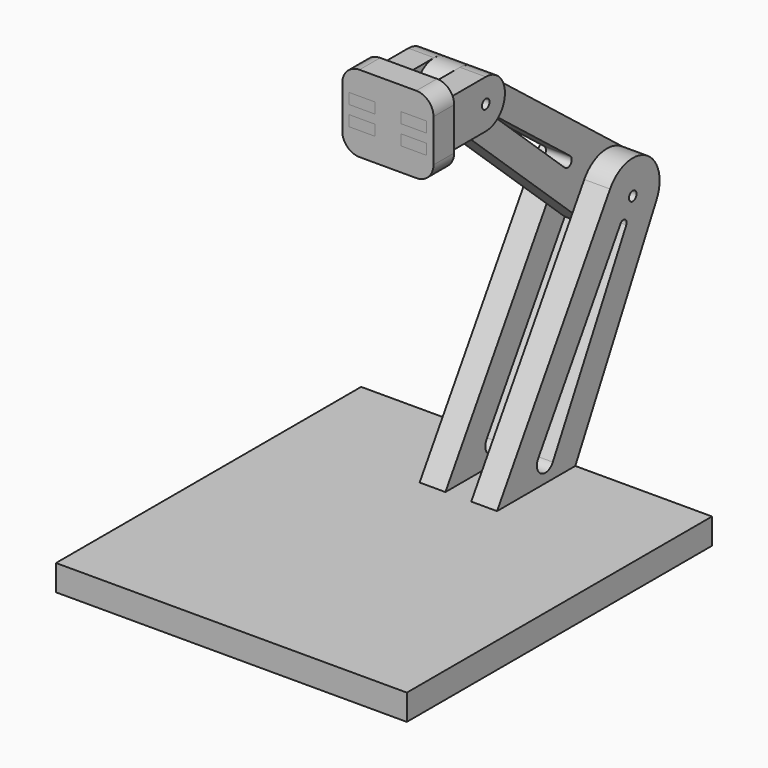
from build123d import *

# Parameters (mm, degrees)
F1_W      = 258.9819133282
F1_H      = 281.5590798855
F2_DEPTH  = 19.05
F4_R      = 3.4925
F5_DEPTH  = 19.05
F7_R      = 3.4925
F8_DEPTH  = 19.05
F9_R      = 3.4925
F10_DEPTH = 19.05
F11_W     = 19.05
F11_H     = 7.8599496324
F12_DEPTH = 19.05
F14_W     = 67.3306509852
F14_H     = 56.7641787347
F15_DEPTH = 19.05
F16_R     = 12.7


# Not quite as in the source:
# - a length typed as a fraction of an inch, garbled in the dataset ("3 / 203.2 mm" for 3/8 in), is restored


with BuildPart() as f2:
    # F1 (on Top) → F2 (new body)
    with BuildSketch(Plane.XY):
        Rectangle(F1_W, F1_H)
    extrude(amount=F2_DEPTH)


with BuildPart() as f5:
    # F4 (on offset) → F5 (new body)
    with BuildSketch(Plane.YZ.offset(9.525)):
        with BuildLine():
            Line((172.8715040576, 185.9790129475), (68.581538884, 19.05))
            Line((68.581538884, 19.05), (140.7795399427, 19.05))
            Line((140.7795399427, 19.05), (215.6994648239, 161.3726968817))
            ThreePointArc((215.6994648239, 161.3726968817), (206.1423956156, 194.3131305331), (172.8715040576, 185.9790129475))
        make_face()
        with BuildLine():
            Line((106.5350997704, 37.813880341), (182.5920726412, 159.5524904553))
            ThreePointArc((182.5920726412, 159.5524904553), (186.6956178335, 160.572252657), (187.8510267574, 156.5048175547))
            Line((187.8510267574, 156.5048175547), (120.0389151124, 29.9881394879))
            ThreePointArc((120.0389151124, 29.9881394879), (109.2420284863, 26.9211405451), (106.5350997704, 37.813880341))
        make_face(mode=Mode.SUBTRACT)
        with Locations((193.8308401065, 172.8845341148)):
            Circle(F4_R, mode=Mode.SUBTRACT)
    extrude(amount=F5_DEPTH)


with BuildPart() as f6_1:
    # F6: instance of F5
    add(f5.part.mirror(Plane.YZ))


with BuildPart() as f8:
    # F7 (on face) → F8 (new body)
    with BuildSketch(Plane.YZ.offset(-9.525)):
        with BuildLine():
            Line((46.176193297, 274.7309380486), (177.1296344703, 154.6683634467))
            ThreePointArc((177.1296344703, 154.6683634467), (212.6905081368, 156.9135583995), (209.0468139458, 192.3584470147))
            Line((209.0468139458, 192.3584470147), (69.05164406, 301.7439030123))
            ThreePointArc((69.05164406, 301.7439030123), (44.6291956916, 299.2333031282), (46.176193297, 274.7309380486))
        make_face()
        with Locations((193.8308401065, 172.8845341148)):
            Circle(F7_R, mode=Mode.SUBTRACT)
        with BuildLine():
            ThreePointArc((86.2107777334, 263.8706501543), (86.2007704818, 264.0291515835), (86.3587549441, 264.0453922064))
            Line((86.3587549441, 264.0453922064), (159.8745879565, 206.6036752981))
            ThreePointArc((159.8745879565, 206.6036752981), (160.4335278853, 201.1664562348), (154.9785168029, 200.8220450298))
            Line((154.9785168029, 200.8220450298), (86.2107777334, 263.8706501543))
        make_face(mode=Mode.SUBTRACT)
        with Locations((58.1461609912, 287.7867005582)):
            Circle(F7_R, mode=Mode.SUBTRACT)
    extrude(amount=F8_DEPTH)


with BuildPart() as f10:
    # F9 (on face) → F10 (new body)
    with BuildSketch(Plane(origin=(-9.525, 0, 0), x_dir=(0, -1, 0), z_dir=(-1, 0, 0))):
        with BuildLine():
            Line((-22.6510197505, 305.4992119924), (-58.1461609912, 305.4992119924))
            ThreePointArc((-58.1461609912, 305.4992119924), (-75.8586724255, 287.7867005582), (-58.1461609912, 270.074189124))
            Line((-58.1461609912, 270.074189124), (-22.6510197505, 270.074189124))
            Line((-22.6510197505, 270.074189124), (-22.6510197505, 305.4992119924))
        make_face()
        with Locations((-58.1461609912, 287.7867005582)):
            Circle(F9_R, mode=Mode.SUBTRACT)
    extrude(amount=F10_DEPTH)

    # F11 (on face) → F12 (join)
    with BuildSketch(Plane.XZ.offset(-22.6510197505)):
        with Locations((-19.05, 295.0008626417)):
            Rectangle(F11_W, F11_H)
        with Locations((-19.05, 280.5725384747)):
            Rectangle(F11_W, F11_H)
    extrude(amount=F12_DEPTH)


with BuildPart() as f13_1:
    # F13: instance of F10
    add(f10.part.mirror(Plane.YZ))


with BuildPart() as f15:
    # F14 (on face) → F15 (new body)
    with BuildSketch(Plane.XZ.offset(-22.6510197505)):
        with Locations((0, 287.7867005582)):
            Rectangle(F14_W, F14_H)
    extrude(amount=F15_DEPTH)

    # F16
    f16_edges = [f15.edges().sort_by_distance(p)[0] for p in [
        (-33.665325, 13.12602, 316.16879),
        (33.665325, 13.12602, 316.16879),
        (33.665325, 13.12602, 259.404611),
        (-33.665325, 13.12602, 259.404611),
    ]]
    fillet(f16_edges, radius=F16_R)

    # F17: cut F10, F13_1
    add(f10.part, mode=Mode.SUBTRACT)
    add(f13_1.part, mode=Mode.SUBTRACT)


solid = Compound([f2.part, f5.part, f6_1.part, f8.part, f10.part, f13_1.part, f15.part])
